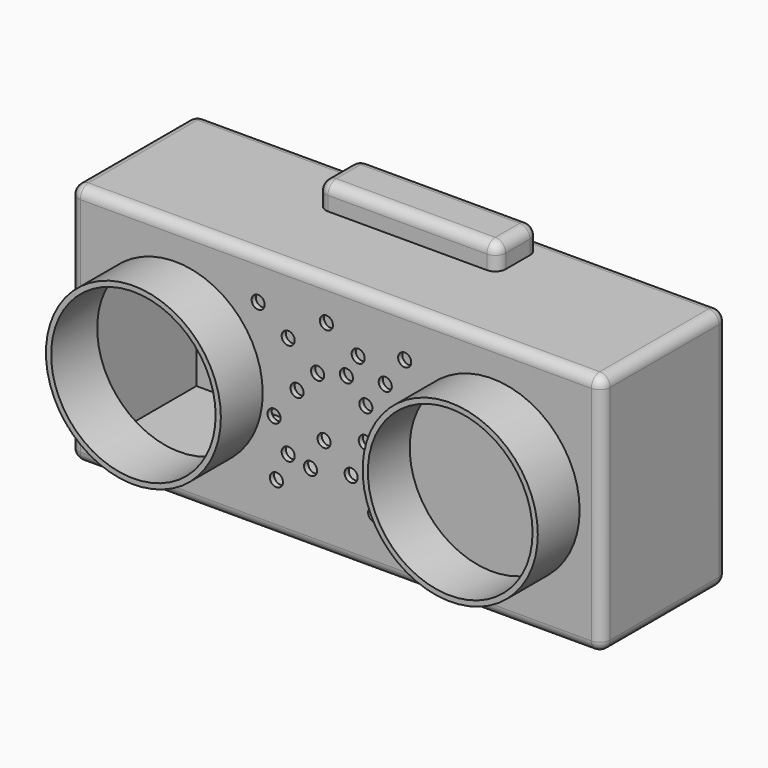
from build123d import *

# Parameters (mm, degrees)
F0_W        = 258.2719624043
F0_H        = 118.0609464645
F1_DEPTH    = 76.2
F2_R        = 42.468670908
F3_DEPTH    = 25.4
F4_T        = -2.54
F5_R        = 42.5232314901
F6_DEPTH    = 25.4
F7_T        = 2.54
F7_T3_DEPTH = 76.2
F7_T5_DEPTH = 258.2719624043
F7_T7_DEPTH = 118.0609464645
F8_W        = 87.3291939497
F8_H        = 24.8894710094
F9_DEPTH    = 11.938
F10_R       = 5.08
F12_D       = 6.35
F14_D       = 6.35


# Not quite as in the source:
# - a shell that OpenCascade refuses in one call is made with other operations: the cavity is built on its own and cut out


with BuildPart() as f1:
    # F0 (on Front) → F1 (new body)
    with BuildSketch(Plane.XZ):
        Rectangle(F0_W, F0_H)
    extrude(amount=F1_DEPTH)

    # F2 (on face) → F3 (join)
    with BuildSketch(Plane.XZ.offset(76.2)):
        with Locations((-77.9456719756, 0)):
            Circle(F2_R)
    extrude(amount=F3_DEPTH)

    # F4
    f4_openings = [f1.faces().sort_by_distance(p)[0] for p in [
        (-77.945672, -101.6, 0),
    ]]
    offset(amount=F4_T, openings=f4_openings, kind=Kind.INTERSECTION)

    # F5 (on face) → F6 (join)
    with BuildSketch(Plane.XZ.offset(76.2)):
        with Locations((75.858682394, 0)):
            Circle(F5_R)
    extrude(amount=F6_DEPTH)

    # F7: shell of thickness 2.54, made by hand


with BuildPart() as f7_core1:
    # F7_t2: copy of F1
    add(f1.part)

    # the walls: a layer under each face that stays
    f7_faces = [f7_core1.faces().sort_by_distance(p)[0] for p in [
        (0, -38.1, 56.4904732323),
        (126.5959812021, -38.1, 0),
        (0, -73.66, 0),
        (-126.5959812021, -38.1, 0),
        (0, -2.54, 0),
        (0, -38.1, -56.4904732323),
        (-117.8743428837, -87.63, 0),
        (-106.2581192476, -101.6, -28.312447272),
        (-120.4143428837, -88.9, 0),
        (0, -76.2, 0),
        (0, -38.1, 59.0304732323),
        (129.1359812021, -38.1, 0),
        (-129.1359812021, -38.1, 0),
        (0, -38.1, -59.0304732323),
        (33.3354509039, -88.9, 0),
        (0, 0, 0),
    ]]
    thicken(f7_faces, amount=-F7_T, mode=Mode.SUBTRACT)

    # F7_s4 → F7_t3 (cut)
    with BuildSketch(Plane.XZ):
        Polygon((126.5705812021, 56.4650732323), (126.5959812021, 59.0304732323), (129.1359812021, 59.0304732323), (129.1359812021, 56.4904732323), align=None)
        Polygon((-126.5705812021, 56.4650732323), (-126.5959812021, 59.0304732323), (-129.1359812021, 59.0304732323), (-129.1359812021, 56.4904732323), align=None)
        Polygon((126.5705812021, -56.4650732323), (129.1359812021, -56.4904732323), (129.1359812021, -59.0304732323), (126.5959812021, -59.0304732323), align=None)
        Polygon((-126.5705812021, -56.4650732323), (-129.1359812021, -56.4904732323), (-129.1359812021, -59.0304732323), (-126.5959812021, -59.0304732323), align=None)
    extrude(amount=F7_T3_DEPTH, mode=Mode.SUBTRACT)

    # F7_s6 → F7_t5 (cut)
    with BuildSketch(Plane.YZ.offset(-129.1359812021)):
        Polygon((-73.6346, 56.4650732323), (-73.66, 59.0304732323), (-76.2, 59.0304732323), (-76.2, 56.4904732323), align=None)
        Polygon((-2.5654, 56.4650732323), (-2.54, 59.0304732323), (0, 59.0304732323), (0, 56.4904732323), align=None)
        Polygon((-73.6346, -56.4650732323), (-76.2, -56.4904732323), (-76.2, -59.0304732323), (-73.66, -59.0304732323), align=None)
        Polygon((-2.5654, -56.4650732323), (0, -56.4904732323), (0, -59.0304732323), (-2.54, -59.0304732323), align=None)
    extrude(amount=F7_T5_DEPTH, mode=Mode.SUBTRACT)

    # F7_s8 → F7_t7 (cut)
    with BuildSketch(Plane.XY.offset(-59.0304732323)):
        Polygon((126.5705812021, -73.6346), (129.1359812021, -73.66), (129.1359812021, -76.2), (126.5959812021, -76.2), align=None)
        Polygon((126.5705812021, -2.5654), (129.1359812021, -2.54), (129.1359812021, 0), (126.5959812021, 0), align=None)
        Polygon((-126.5705812021, -73.6346), (-126.5959812021, -76.2), (-129.1359812021, -76.2), (-129.1359812021, -73.66), align=None)
        Polygon((-126.5705812021, -2.5654), (-129.1359812021, -2.54), (-129.1359812021, 0), (-126.5959812021, 0), align=None)
    extrude(amount=F7_T7_DEPTH, mode=Mode.SUBTRACT)

    # F7_s9 → F7_t10 (revolve, cut)
    with BuildSketch(Plane.XY):
        Polygon((-35.4516010676, -76.2254), (-38.0170010676, -76.2), (-38.0170010676, -73.66), (-35.4770010676, -73.66), align=None)
    revolve(axis=Axis((-77.9456719756, -76.2, 0), (0, -1, 0)), mode=Mode.SUBTRACT)

    # F7_s11 → F7_t12 (revolve, cut)
    with BuildSketch(Plane.XY):
        Polygon((118.4073138841, -76.2254), (118.3819138841, -73.66), (115.8419138841, -73.66), (115.8419138841, -76.2), align=None)
    revolve(axis=Axis((75.858682394, -76.2, 0), (0, -1, 0)), mode=Mode.SUBTRACT)


with BuildPart() as f1_1:
    add(f1.part)

    # what is left inside the walls is the cavity
    f7_cavity = [f7_core1.part.solids().sort_by_distance(p)[0] for p in [
        (35.900851, -93.133333, 0),
    ]]
    add(f7_cavity, mode=Mode.SUBTRACT)

    # F8 (on face) → F9 (join)
    with BuildSketch(Plane.XY.offset(59.0304732323)):
        with Locations((0, -20.2801432461)):
            Rectangle(F8_W, F8_H)
    extrude(amount=F9_DEPTH)

    # F10
    f10_edges = [f1_1.edges().sort_by_distance(p)[0] for p in [
        (-129.135981, -38.1, 59.030473),
        (-129.135981, -38.1, -59.030473),
        (129.135981, -38.1, 59.030473),
        (129.135981, -38.1, -59.030473),
        (129.135981, -76.2, 0),
        (0, -76.2, 59.030473),
        (0, -76.2, -59.030473),
        (129.135981, 0, 0),
        (0, 0, 59.030473),
        (0, 0, -59.030473),
        (-129.135981, 0, 0),
        (-129.135981, -76.2, 0),
        (-43.664597, -20.280143, 70.968473),
        (0, -32.724879, 70.968473),
        (0, -7.835408, 70.968473),
        (43.664597, -20.280143, 70.968473),
        (-43.664597, -32.724879, 64.999473),
        (-43.664597, -7.835408, 64.999473),
        (43.664597, -32.724879, 64.999473),
        (43.664597, -7.835408, 64.999473),
    ]]
    fillet(f10_edges, radius=F10_R)

    # F12 (through all)
    with Locations(Plane.XZ.offset(76.2)):
        with Locations((-4.5539974235, 40.1396788657)):
            Hole(F12_D / 2)

    # F14 (through all)
    with Locations(Plane.XZ.offset(76.2)):
        with Locations((-37.6857295632, 38.1780304015), (-23.1191907078, 27.56604366), (10.8693959191, 30.9581160545), (33.4332510829, 36.6552881896), (24.007840082, 23.2110135257), (-8.8382726535, 17.2407273203), (5.1570278592, 20.6584427506), (-18.8349168748, 6.6602416337), (14.5824337378, 10.9119648114), (27.149643749, 3.7382091396), (24.007840082, -15.726538375), (14.2968157306, -4.8344726674), (-29.9740321934, -7.9270545393), (-5.6964703836, -10.5349421501), (-23.1191907078, -21.9648182392), (-12.2656933963, -24.5554894209), (-28.8315601647, -34.8412431777), (7.4419751763, -21.1450979114), (18.8667103648, -34.3298055232)):
            Hole(F14_D / 2)


solid = f1_1.part
